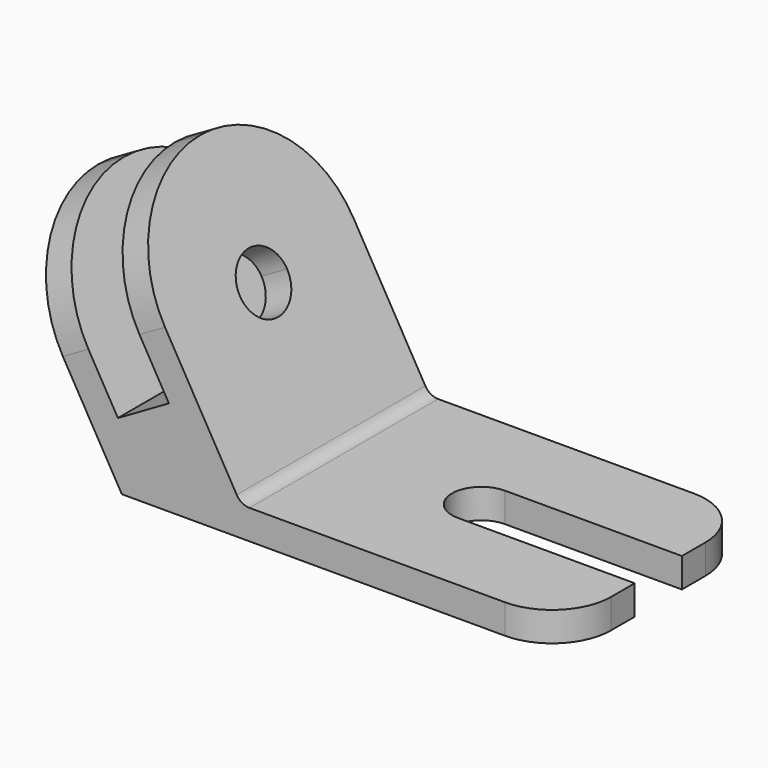
from build123d import *

# Parameters (mm, degrees)
F1_DEPTH = 80
F3_DEPTH = 27.9
F4_R     = 20
F6_R     = 39.99999
F7_R     = 5
F8_DEPTH = 148.2


# Not quite as in the source:
# - a fillet or chamfer is up to 0.001 mm smaller than in the source, because OpenCascade refuses the exact size


with BuildPart() as f1:
    # F0 (on Front) → F1 (new body)
    with BuildSketch(Plane.XZ):
        Polygon((-150, 0), (0, 0), (0, 10), (-109.5854811567, 10), (-155.3589838486, 89.2820323028), (-164.0192378865, 84.2820323028), (-134.0192378865, 32.3205080757), (-151.3397459622, 22.3205080757), (-181.3397459622, 74.2820323028), (-190, 69.2820323028), align=None)
    extrude(amount=F1_DEPTH)

    # F2 (on Top) → F3 (cut)
    with BuildSketch(Plane.XY):
        with BuildLine():
            Line((-60, -40), (-60, -30))
            ThreePointArc((-60, -30), (-70, -40), (-60, -50))
            Line((-60, -50), (-60, -40))
        make_face()
        with BuildLine():
            ThreePointArc((-50, -40), (-52.9289321881, -32.9289321881), (-60, -30))
            Line((-60, -30), (-60, -40))
            Line((-60, -40), (-50, -40))
        make_face()
        with BuildLine():
            ThreePointArc((-60, -50), (-52.9289321881, -47.0710678119), (-50, -40))
            Line((-50, -40), (-60, -40))
            Line((-60, -40), (-60, -50))
        make_face()
        with BuildLine():
            Line((0, -50), (0, -40))
            Line((0, -40), (-50, -40))
            ThreePointArc((-50, -40), (-52.9289321881, -47.0710678119), (-60, -50))
            Line((-60, -50), (0, -50))
        make_face()
        with BuildLine():
            Line((0, -40), (0, -30))
            Line((0, -30), (-60, -30))
            ThreePointArc((-60, -30), (-52.9289321881, -32.9289321881), (-50, -40))
            Line((-50, -40), (0, -40))
        make_face()
    extrude(amount=F3_DEPTH, mode=Mode.SUBTRACT)

    # F4
    f4_edges = [f1.edges().sort_by_distance(p)[0] for p in [
        (0, 0, 5),
        (0, -80, 5),
    ]]
    fillet(f4_edges, radius=F4_R)

    # F6 (radius 40 in the source; OpenCascade refuses exactly that, so slightly less here)
    f6_edges = [f1.edges().sort_by_distance(p)[0] for p in [
        (-159.689111, 0, 86.782032),
        (-185.669873, 0, 71.782032),
        (-185.669873, -80, 71.782032),
        (-159.689111, -80, 86.782032),
    ]]
    fillet(f6_edges, radius=F6_R)

    # F7
    f7_edges = [f1.edges().sort_by_distance(p)[0] for p in [
        (-109.585481, -40, 10),
    ]]
    fillet(f7_edges, radius=F7_R)

    # F5 (on face) → F8 (cut)
    with BuildSketch(Plane(origin=(-77.8589838486, 0, -44.9519052838), x_dir=(0, 1, 0), z_dir=(0.8660254038, 0, 0.5))):
        with BuildLine():
            Line((-40, 112.1529946162), (-40, 102.1529946162))
            ThreePointArc((-40, 102.1529946162), (-32.9289321881, 105.0819268043), (-30, 112.1529946162))
            ThreePointArc((-30, 112.1529946162), (-40, 122.1529946162), (-50, 112.1529946162))
            Line((-50, 112.1529946162), (-40, 112.1529946162))
        make_face()
        with BuildLine():
            ThreePointArc((-50, 112.1529946162), (-47.0710678119, 105.0819268043), (-40, 102.1529946162))
            Line((-40, 102.1529946162), (-40, 112.1529946162))
            Line((-40, 112.1529946162), (-50, 112.1529946162))
        make_face()
    extrude(amount=-F8_DEPTH, mode=Mode.SUBTRACT)


solid = f1.part
